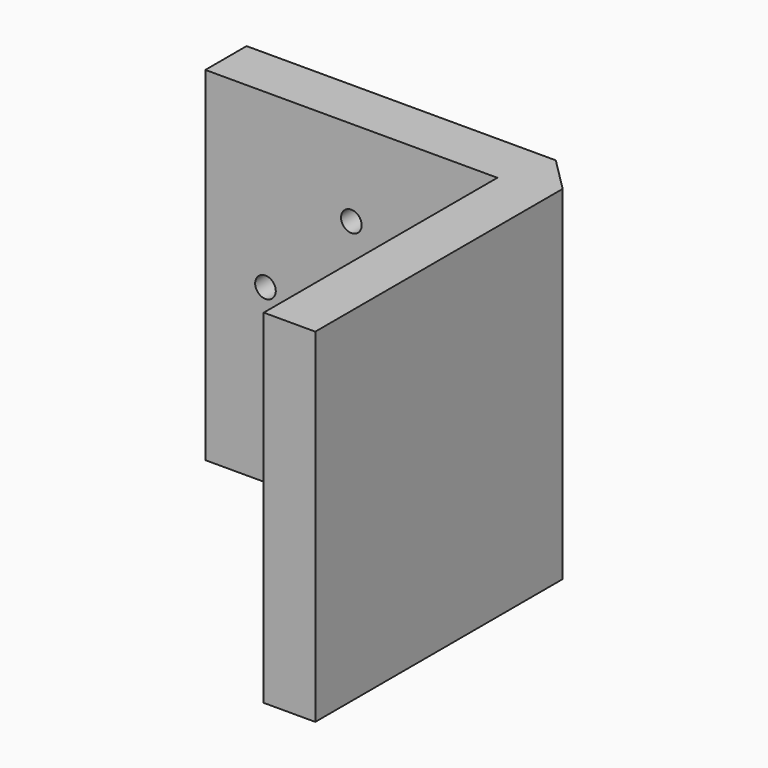
from build123d import *

# Parameters (mm, degrees)
F1_DEPTH        = 10
F2_SIZE         = 2
F4_D            = 1.2
F4_DEPTH        = 4
F4_TIP          = 0.3605163714
F4_COPIES_COUNT = 4


# Not quite as in the source:
# - a pattern or mirror of a feature is missing from the dataset's text; its kind, count and spacing are read off the source's solid


with BuildPart() as f1:
    # F0 (on Top) → F1 (new body, symmetric)
    with BuildSketch(Plane.XY):
        Polygon((8.5, 1.5), (-8.5, 1.5), (-8.5, -1.5), (8.5, -1.5), (8.5, -18.5), (11.5, -18.5), (11.5, 1.5), align=None)
    extrude(amount=F1_DEPTH, both=True)

    # F2
    f2_edges = [f1.edges().sort_by_distance(p)[0] for p in [
        (11.5, 1.5, 0),
    ]]
    chamfer(f2_edges, length=F2_SIZE)

    # F4
    with Locations(Plane.XZ.offset(1.5)):
        with Locations((-5, 0)):
            f4 = Hole(F4_D / 2, depth=F4_DEPTH)
            with Locations((0, 0, -(F4_DEPTH + F4_TIP / 2))):  # 118° drill point
                Cone(0, F4_D / 2, F4_TIP, mode=Mode.SUBTRACT)

    # F4_copies: F4 ×4 about axis
    f4_copies_axis = Axis((0, 0, 0), (0, 1, 0))
    for i in range(1, F4_COPIES_COUNT):
        add(f4.rotate(f4_copies_axis, i * 360 / F4_COPIES_COUNT), mode=Mode.SUBTRACT)


solid = f1.part
